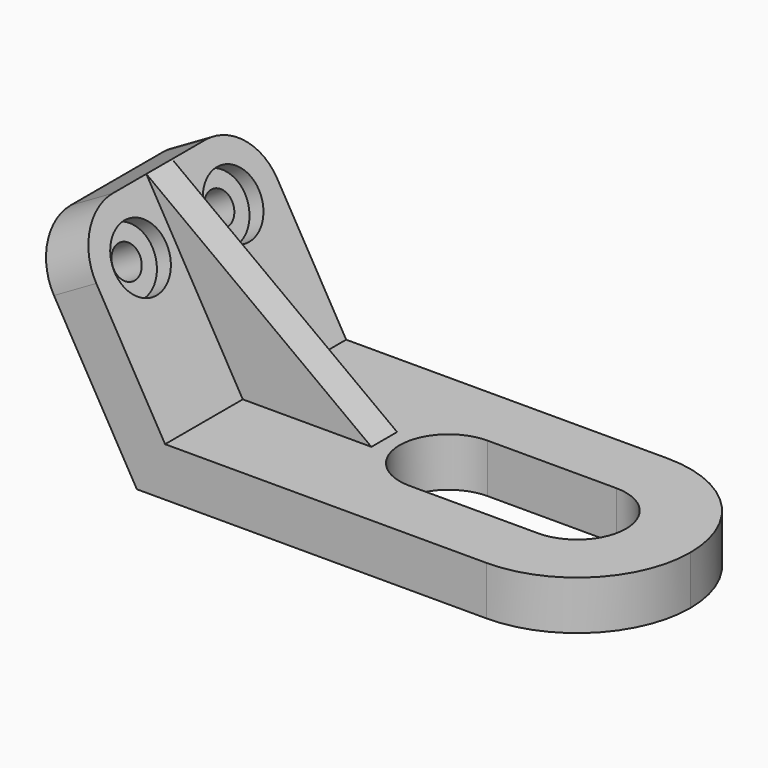
from build123d import *

# Parameters (mm, degrees)
F1_DEPTH = 22.352
F2_DEPTH = 3.175
F3_R     = 22.35199
F5_DEPTH = 9.652
F7_R     = 3.175
F8_DEPTH = 25.4
F7_R_2   = 6.35
F9_DEPTH = 3.175
F10_R    = 10.922


# Not quite as in the source:
# - a fillet or chamfer is up to 0.001 mm smaller than in the source, because OpenCascade refuses the exact size


with BuildPart() as f1:
    # F0 (on Front) → F1 (new body, symmetric)
    with BuildSketch(Plane.XZ):
        Polygon((-21.8362923991, 37.8215678842), (0, 0), (91.4245847982, 0), (91.4245847982, 9.652), (30.9725847982, 9.652), (5.5725847982, 9.652), (-13.4774152018, 42.6475678842), align=None)
    extrude(amount=F1_DEPTH, both=True)

    # F0 (on Front) → F2 (join, symmetric)
    with BuildSketch(Plane.XZ):
        Polygon((30.9725847982, 9.652), (-13.4774152018, 42.6475678842), (5.5725847982, 9.652), align=None)
    extrude(amount=F2_DEPTH, both=True)

    # F3 (radius 22.352 in the source; OpenCascade refuses exactly that, so slightly less here)
    f3_edges = [f1.edges().sort_by_distance(p)[0] for p in [
        (91.424585, 22.352, 4.826),
        (91.424585, -22.352, 4.826),
    ]]
    fillet(f3_edges, radius=F3_R)

    # F4 (on face) → F5 (cut, through all)
    with BuildSketch(Plane.XY.offset(9.652)):
        with BuildLine():
            Line((69.0725847982, 9.652), (43.6725847982, 9.652))
            ThreePointArc((43.6725847982, 9.652), (34.0205847982, 0), (43.6725847982, -9.652))
            Line((43.6725847982, -9.652), (69.0725847982, -9.652))
            ThreePointArc((69.0725847982, -9.652), (78.7245847982, 0), (69.0725847982, 9.652))
        make_face()
    extrude(amount=-F5_DEPTH, mode=Mode.SUBTRACT)

    # F7 (on face) → F8 (cut)
    with BuildSketch(Plane(origin=(8.3588771973, 0, 4.826), x_dir=(0, 1, 0), z_dir=(0.8660254038, 0, 0.5))):
        with Locations((11.43, 32.7505847982)):
            Circle(F7_R)
        with Locations((-11.43, 32.7505847982)):
            Circle(F7_R)
    extrude(amount=-F8_DEPTH, mode=Mode.SUBTRACT)

    # F7 (on face) → F9 (cut)
    with BuildSketch(Plane(origin=(8.3588771973, 0, 4.826), x_dir=(0, 1, 0), z_dir=(0.8660254038, 0, 0.5))):
        with Locations((-11.43, 32.7505847982)):
            Circle(F7_R_2)
        with Locations((-11.43, 32.7505847982)):
            Circle(F7_R, mode=Mode.SUBTRACT)
        with Locations((11.43, 32.7505847982)):
            Circle(F7_R_2)
        with Locations((11.43, 32.7505847982)):
            Circle(F7_R, mode=Mode.SUBTRACT)
    extrude(amount=-F9_DEPTH, mode=Mode.SUBTRACT)

    # F10
    f10_edges = [f1.edges().sort_by_distance(p)[0] for p in [
        (-17.656854, 22.352, 40.234568),
        (-17.656854, -22.352, 40.234568),
    ]]
    fillet(f10_edges, radius=F10_R)


solid = f1.part
